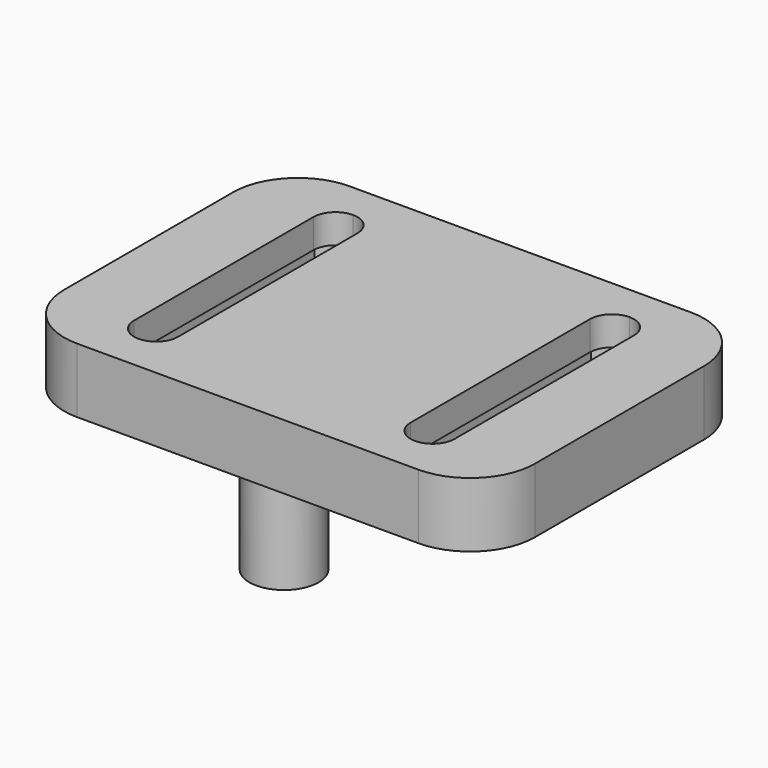
from build123d import *

# Parameters (mm, degrees)
F1_R     = 2.3375
F2_DEPTH = 7.5
F1_R_2   = 2.675
F4_DEPTH = 5
F5_R     = 5
F7_DEPTH = 2.75


# Not quite as in the source:
# - a feature names something its author has since deleted; it is built from what else it names


with BuildPart() as f2:
    # F1 (on Top) → F2 (new body)
    with BuildSketch(Plane.XY):
        with Locations((0, 19.305)):
            Circle(F1_R)
    extrude(amount=F2_DEPTH)



with BuildPart() as f2b:
    # F1 (on Top) → F2, piece 2 (new body)
    with BuildSketch(Plane.XY):
        Circle(F1_R_2)
    extrude(amount=F2_DEPTH)


with BuildPart() as f2_1:
    add(f2.part)

    add(f2b.part)  # F4 merges F2b
    # F3 (on face) → F4 (join)
    with BuildSketch(Plane.XY.offset(7.5)):
        with BuildLine():
            Line((0, 21.6425), (0, 22.805))
            Line((0, 22.805), (-10.675, 22.805))
            Line((-10.675, 22.805), (-10.675, 20.005))
            ThreePointArc((-10.675, 20.005), (-9.472918472, 19.507081528), (-8.975, 18.305))
            Line((-8.975, 18.305), (-8.975, 1))
            ThreePointArc((-8.975, 1), (-9.472918472, -0.202081528), (-10.675, -0.7))
            Line((-10.675, -0.7), (-10.675, -3.5))
            Line((-10.675, -3.5), (0, -3.5))
            Line((0, -3.5), (0, 16.9675))
            ThreePointArc((0, 16.9675), (-2.3375, 19.305), (0, 21.6425))
        make_face()
        with BuildLine():
            Line((10.675, 22.805), (0, 22.805))
            Line((0, 22.805), (0, 21.6425))
            ThreePointArc((0, 21.6425), (1.652862101, 20.957862101), (2.3375, 19.305))
            ThreePointArc((2.3375, 19.305), (1.652862101, 17.652137899), (0, 16.9675))
            Line((0, 16.9675), (0, -3.5))
            Line((0, -3.5), (10.675, -3.5))
            Line((10.675, -3.5), (10.675, -0.7))
            ThreePointArc((10.675, -0.7), (9.472918472, -0.202081528), (8.975, 1))
            Line((8.975, 1), (8.975, 18.305))
            ThreePointArc((8.975, 18.305), (9.472918472, 19.507081528), (10.675, 20.005))
            Line((10.675, 20.005), (10.675, 22.805))
        make_face()
        with BuildLine():
            Line((0, 16.9675), (0, 21.6425))
            ThreePointArc((0, 21.6425), (-2.3375, 19.305), (0, 16.9675))
        make_face()
        with BuildLine():
            ThreePointArc((2.3375, 19.305), (1.652862101, 20.957862101), (0, 21.6425))
            Line((0, 21.6425), (0, 16.9675))
            ThreePointArc((0, 16.9675), (1.652862101, 17.652137899), (2.3375, 19.305))
        make_face()
        with BuildLine():
            Line((-10.675, 20.005), (-10.675, 22.805))
            Line((-10.675, 22.805), (-18.175, 22.805))
            Line((-18.175, 22.805), (-18.175, -3.5))
            Line((-18.175, -3.5), (-10.675, -3.5))
            Line((-10.675, -3.5), (-10.675, -0.7))
            ThreePointArc((-10.675, -0.7), (-11.877081528, -0.202081528), (-12.375, 1))
            Line((-12.375, 1), (-12.375, 18.305))
            ThreePointArc((-12.375, 18.305), (-11.877081528, 19.507081528), (-10.675, 20.005))
        make_face()
        with BuildLine():
            Line((18.175, 22.805), (10.675, 22.805))
            Line((10.675, 22.805), (10.675, 20.005))
            ThreePointArc((10.675, 20.005), (11.877081528, 19.507081528), (12.375, 18.305))
            Line((12.375, 18.305), (12.375, 1))
            ThreePointArc((12.375, 1), (11.877081528, -0.202081528), (10.675, -0.7))
            Line((10.675, -0.7), (10.675, -3.5))
            Line((10.675, -3.5), (18.175, -3.5))
            Line((18.175, -3.5), (18.175, 22.805))
        make_face()
    extrude(amount=F4_DEPTH)

    # F5
    f5_edges = [f2_1.edges().sort_by_distance(p)[0] for p in [
        (-18.175, 22.805, 10),
        (-18.175, -3.5, 10),
        (18.175, -3.5, 10),
        (18.175, 22.805, 10),
    ]]
    fillet(f5_edges, radius=F5_R)

    # F6 (on face) → F7 (cut)
    with BuildSketch(Plane(origin=(0, 0, 7.5), x_dir=(1, 0, 0), z_dir=(0, 0, -1))):
        Polygon((-7.675, 0.7320508076), (-10.675, 2.4641016151), (-13.675, 0.7320508076), (-13.675, -2.7320508076), (-10.675, -4.4641016151), (-7.675, -2.7320508076), align=None)
        Polygon((-7.675, -16.5729491924), (-7.675, -2.7320508076), (-10.675, -4.4641016151), (-13.675, -2.7320508076), (-13.675, -16.5729491924), (-10.675, -14.8408983849), align=None)
        Polygon((-7.675, -20.0370508076), (-7.675, -16.5729491924), (-10.675, -14.8408983849), (-13.675, -16.5729491924), (-13.675, -20.0370508076), (-10.675, -21.7691016151), align=None)
        Polygon((10.675, 2.4641016151), (7.675, 0.7320508076), (7.675, -2.7320508076), (10.675, -4.4641016151), (13.675, -2.7320508076), (13.675, 0.7320508076), align=None)
        Polygon((10.675, -4.4641016151), (7.675, -2.7320508076), (7.675, -16.5729491924), (10.675, -14.8408983849), (13.675, -16.5729491924), (13.675, -2.7320508076), align=None)
        Polygon((10.675, -14.8408983849), (7.675, -16.5729491924), (7.675, -20.0370508076), (10.675, -21.7691016151), (13.675, -20.0370508076), (13.675, -16.5729491924), align=None)
    extrude(amount=-F7_DEPTH, mode=Mode.SUBTRACT)


solid = f2_1.part
